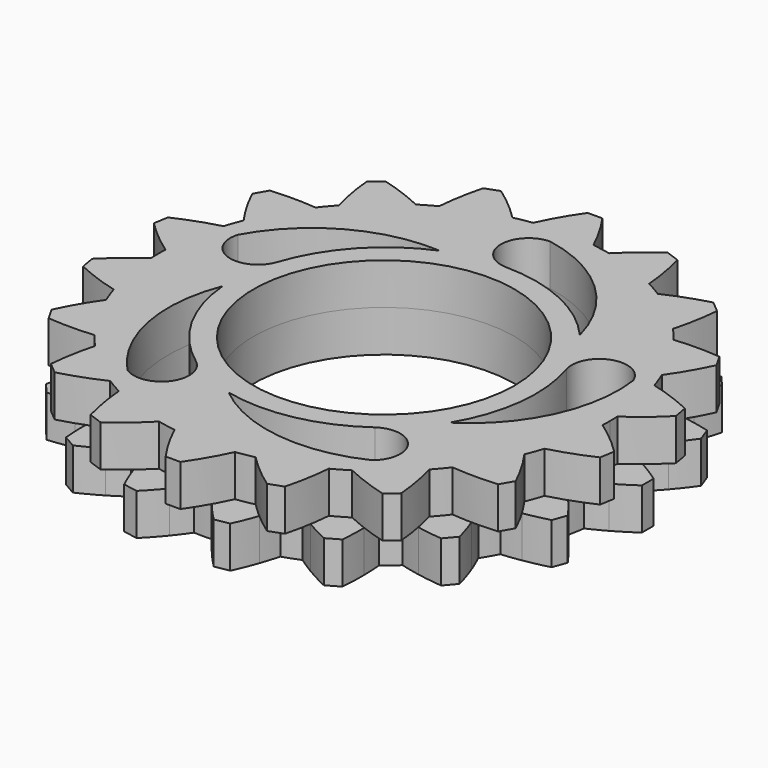
from build123d import *

# Parameters (mm, degrees)
F0_R     = 10.9982
F1_DEPTH = 3.5
F2_R     = 10.9982
F3_DEPTH = 3.5
F5_DEPTH = 25.4


with BuildPart() as f1:
    # F0 (on Top) → F1 (new body)
    with BuildSketch(Plane.XY):
        with BuildLine():
            ThreePointArc((-8.8441278606, 16.8725784154), (-6.5154837304, 17.901144426), (-4.070489347, 18.6100407435))
            ThreePointArc((-4.070489347, 18.6100407435), (-5.4892281389, 19.919494063), (-7.0197279531, 21.0963789657))
            Line((-7.0197279531, 21.0963789657), (-8.1830674177, 20.6729580282))
            ThreePointArc((-8.1830674177, 20.6729580282), (-8.5990112621, 18.7876255712), (-8.8441278606, 16.8725784154))
        make_face()
        with BuildLine():
            ThreePointArc((19.0341454654, -0.7770498061), (19.0460359539, -0.3886057666), (19.05, 0))
            ThreePointArc((19.05, 0), (19.0460359539, 0.3886057666), (19.0341454654, 0.7770498061))
            ThreePointArc((19.0341454654, 0.7770498061), (18.7605876949, 3.3079977846), (18.1520127229, 5.7798731914))
            ThreePointArc((18.1520127229, 5.7798731914), (17.901144426, 6.5154837304), (17.6204793508, 7.2402491289))
            ThreePointArc((17.6204793508, 7.2402491289), (16.4977839421, 9.525), (15.0804793508, 11.6396581802))
            ThreePointArc((15.0804793508, 11.6396581802), (14.5931466414, 12.2451039645), (14.0815233758, 12.8301675521))
            ThreePointArc((14.0815233758, 12.8301675521), (12.2451039645, 14.5931466414), (10.1900176048, 16.0955286093))
            ThreePointArc((10.1900176048, 16.0955286093), (9.525, 16.4977839421), (8.8441278606, 16.8725784154))
            ThreePointArc((8.8441278606, 16.8725784154), (6.5154837304, 17.901144426), (4.070489347, 18.6100407435))
            ThreePointArc((4.070489347, 18.6100407435), (3.3079977846, 18.7605876949), (2.54, 18.8799073091))
            ThreePointArc((2.54, 18.8799073091), (0, 19.05), (-2.54, 18.8799073091))
            ThreePointArc((-2.54, 18.8799073091), (-3.3079977846, 18.7605876949), (-4.070489347, 18.6100407435))
            ThreePointArc((-4.070489347, 18.6100407435), (-6.5154837304, 17.901144426), (-8.8441278606, 16.8725784154))
            ThreePointArc((-8.8441278606, 16.8725784154), (-9.525, 16.4977839421), (-10.1900176048, 16.0955286093))
            ThreePointArc((-10.1900176048, 16.0955286093), (-12.2451039645, 14.5931466414), (-14.0815233758, 12.8301675521))
            ThreePointArc((-14.0815233758, 12.8301675521), (-14.5931466414, 12.2451039645), (-15.0804793508, 11.6396581802))
            ThreePointArc((-15.0804793508, 11.6396581802), (-16.4977839421, 9.525), (-17.6204793508, 7.2402491289))
            ThreePointArc((-17.6204793508, 7.2402491289), (-17.901144426, 6.5154837304), (-18.1520127229, 5.7798731914))
            ThreePointArc((-18.1520127229, 5.7798731914), (-18.7605876949, 3.3079977846), (-19.0341454654, 0.7770498061))
            ThreePointArc((-19.0341454654, 0.7770498061), (-19.05, 0), (-19.0341454654, -0.7770498061))
            ThreePointArc((-19.0341454654, -0.7770498061), (-18.7605876949, -3.3079977846), (-18.1520127229, -5.7798731914))
            ThreePointArc((-18.1520127229, -5.7798731914), (-17.901144426, -6.5154837304), (-17.6204793508, -7.2402491289))
            ThreePointArc((-17.6204793508, -7.2402491289), (-16.4977839421, -9.525), (-15.0804793508, -11.6396581802))
            ThreePointArc((-15.0804793508, -11.6396581802), (-14.5931466414, -12.2451039645), (-14.0815233758, -12.8301675521))
            ThreePointArc((-14.0815233758, -12.8301675521), (-12.2451039645, -14.5931466414), (-10.1900176048, -16.0955286093))
            ThreePointArc((-10.1900176048, -16.0955286093), (-9.525, -16.4977839421), (-8.8441278606, -16.8725784154))
            ThreePointArc((-8.8441278606, -16.8725784154), (-6.5154837304, -17.901144426), (-4.070489347, -18.6100407435))
            ThreePointArc((-4.070489347, -18.6100407435), (-3.3079977846, -18.7605876949), (-2.54, -18.8799073091))
            ThreePointArc((-2.54, -18.8799073091), (0, -19.05), (2.54, -18.8799073091))
            ThreePointArc((2.54, -18.8799073091), (3.3079977846, -18.7605876949), (4.070489347, -18.6100407435))
            ThreePointArc((4.070489347, -18.6100407435), (6.5154837304, -17.901144426), (8.8441278606, -16.8725784154))
            ThreePointArc((8.8441278606, -16.8725784154), (9.525, -16.4977839421), (10.1900176048, -16.0955286093))
            ThreePointArc((10.1900176048, -16.0955286093), (12.2451039645, -14.5931466414), (14.0815233758, -12.8301675521))
            ThreePointArc((14.0815233758, -12.8301675521), (14.5931466414, -12.2451039645), (15.0804793508, -11.6396581802))
            ThreePointArc((15.0804793508, -11.6396581802), (16.4977839421, -9.525), (17.6204793508, -7.2402491289))
            ThreePointArc((17.6204793508, -7.2402491289), (17.901144426, -6.5154837304), (18.1520127229, -5.7798731914))
            ThreePointArc((18.1520127229, -5.7798731914), (18.7605876949, -3.3079977846), (19.0341454654, -0.7770498061))
        make_face()
        Circle(F0_R, mode=Mode.SUBTRACT)
        with BuildLine():
            ThreePointArc((-2.54, 18.8799073091), (0, 19.05), (2.54, 18.8799073091))
            ThreePointArc((2.54, 18.8799073091), (1.6546810385, 20.5956281756), (0.619, 22.225))
            Line((0.619, 22.225), (-0.619, 22.225))
            ThreePointArc((-0.619, 22.225), (-1.6546810385, 20.5956281756), (-2.54, 18.8799073091))
        make_face()
        with BuildLine():
            ThreePointArc((4.070489347, 18.6100407435), (6.5154837304, 17.901144426), (8.8441278606, 16.8725784154))
            ThreePointArc((8.8441278606, 16.8725784154), (8.5990112621, 18.7876255712), (8.1830674177, 20.6729580282))
            Line((8.1830674177, 20.6729580282), (7.0197279531, 21.0963789657))
            ThreePointArc((7.0197279531, 21.0963789657), (5.4892281389, 19.919494063), (4.070489347, 18.6100407435))
        make_face()
        with BuildLine():
            ThreePointArc((10.1900176048, 16.0955286093), (12.2451039645, 14.5931466414), (14.0815233758, 12.8301675521))
            ThreePointArc((14.0815233758, 12.8301675521), (14.5061738197, 14.713558047), (14.7601361356, 16.6274522179))
            Line((14.7601361356, 16.6274522179), (13.811773115, 17.4232232787))
            ThreePointArc((13.811773115, 17.4232232787), (11.9710553903, 16.840774986), (10.1900176048, 16.0955286093))
        make_face()
        with BuildLine():
            ThreePointArc((15.0804793508, 11.6396581802), (16.4977839421, 9.525), (17.6204793508, 7.2402491289))
            ThreePointArc((17.6204793508, 7.2402491289), (18.6636777262, 8.8648182733), (19.5569145991, 10.5764302751))
            Line((19.5569145991, 10.5764302751), (18.9379145991, 11.6485697249))
            ThreePointArc((18.9379145991, 11.6485697249), (17.0089966878, 11.7308099023), (15.0804793508, 11.6396581802))
        make_face()
        with BuildLine():
            ThreePointArc((18.1520127229, 5.7798731914), (18.7605876949, 3.3079977846), (19.0341454654, 0.7770498061))
            ThreePointArc((19.0341454654, 0.7770498061), (20.5700666525, 1.9468505852), (21.9948405327, 3.2497347495))
            Line((21.9948405327, 3.2497347495), (21.7798640887, 4.4689267478))
            ThreePointArc((21.7798640887, 4.4689267478), (19.9954019586, 5.2059360161), (18.1520127229, 5.7798731914))
        make_face()
        with BuildLine():
            ThreePointArc((21.9948405327, -3.2497347495), (20.5700666525, -1.9468505852), (19.0341454654, -0.7770498061))
            ThreePointArc((19.0341454654, -0.7770498061), (18.7605876949, -3.3079977846), (18.1520127229, -5.7798731914))
            ThreePointArc((18.1520127229, -5.7798731914), (19.9954019586, -5.2059360161), (21.7798640887, -4.4689267478))
            Line((21.7798640887, -4.4689267478), (21.9948405327, -3.2497347495))
        make_face()
        with BuildLine():
            ThreePointArc((19.5569145991, -10.5764302751), (18.6636777262, -8.8648182733), (17.6204793508, -7.2402491289))
            ThreePointArc((17.6204793508, -7.2402491289), (16.4977839421, -9.525), (15.0804793508, -11.6396581802))
            ThreePointArc((15.0804793508, -11.6396581802), (17.0089966878, -11.7308099023), (18.9379145991, -11.6485697249))
            Line((18.9379145991, -11.6485697249), (19.5569145991, -10.5764302751))
        make_face()
        with BuildLine():
            ThreePointArc((14.7601361356, -16.6274522179), (14.5061738197, -14.713558047), (14.0815233758, -12.8301675521))
            ThreePointArc((14.0815233758, -12.8301675521), (12.2451039645, -14.5931466414), (10.1900176048, -16.0955286093))
            ThreePointArc((10.1900176048, -16.0955286093), (11.9710553903, -16.840774986), (13.811773115, -17.4232232787))
            Line((13.811773115, -17.4232232787), (14.7601361356, -16.6274522179))
        make_face()
        with BuildLine():
            ThreePointArc((8.1830674177, -20.6729580282), (8.5990112621, -18.7876255712), (8.8441278606, -16.8725784154))
            ThreePointArc((8.8441278606, -16.8725784154), (6.5154837304, -17.901144426), (4.070489347, -18.6100407435))
            ThreePointArc((4.070489347, -18.6100407435), (5.4892281389, -19.919494063), (7.0197279531, -21.0963789657))
            Line((7.0197279531, -21.0963789657), (8.1830674177, -20.6729580282))
        make_face()
        with BuildLine():
            ThreePointArc((0.619, -22.225), (1.6546810385, -20.5956281756), (2.54, -18.8799073091))
            ThreePointArc((2.54, -18.8799073091), (0, -19.05), (-2.54, -18.8799073091))
            ThreePointArc((-2.54, -18.8799073091), (-1.6546810385, -20.5956281756), (-0.619, -22.225))
            Line((-0.619, -22.225), (0.619, -22.225))
        make_face()
        with BuildLine():
            ThreePointArc((-7.0197279531, -21.0963789657), (-5.4892281389, -19.919494063), (-4.070489347, -18.6100407435))
            ThreePointArc((-4.070489347, -18.6100407435), (-6.5154837304, -17.901144426), (-8.8441278606, -16.8725784154))
            ThreePointArc((-8.8441278606, -16.8725784154), (-8.5990112621, -18.7876255712), (-8.1830674177, -20.6729580282))
            Line((-8.1830674177, -20.6729580282), (-7.0197279531, -21.0963789657))
        make_face()
        with BuildLine():
            ThreePointArc((-13.811773115, -17.4232232787), (-11.9710553903, -16.840774986), (-10.1900176048, -16.0955286093))
            ThreePointArc((-10.1900176048, -16.0955286093), (-12.2451039645, -14.5931466414), (-14.0815233758, -12.8301675521))
            ThreePointArc((-14.0815233758, -12.8301675521), (-14.5061738197, -14.713558047), (-14.7601361356, -16.6274522179))
            Line((-14.7601361356, -16.6274522179), (-13.811773115, -17.4232232787))
        make_face()
        with BuildLine():
            ThreePointArc((-18.9379145991, -11.6485697249), (-17.0089966878, -11.7308099023), (-15.0804793508, -11.6396581802))
            ThreePointArc((-15.0804793508, -11.6396581802), (-16.4977839421, -9.525), (-17.6204793508, -7.2402491289))
            ThreePointArc((-17.6204793508, -7.2402491289), (-18.6636777262, -8.8648182733), (-19.5569145991, -10.5764302751))
            Line((-19.5569145991, -10.5764302751), (-18.9379145991, -11.6485697249))
        make_face()
        with BuildLine():
            ThreePointArc((-21.7798640887, -4.4689267478), (-19.9954019586, -5.2059360161), (-18.1520127229, -5.7798731914))
            ThreePointArc((-18.1520127229, -5.7798731914), (-18.7605876949, -3.3079977846), (-19.0341454654, -0.7770498061))
            ThreePointArc((-19.0341454654, -0.7770498061), (-20.5700666525, -1.9468505852), (-21.9948405327, -3.2497347495))
            Line((-21.9948405327, -3.2497347495), (-21.7798640887, -4.4689267478))
        make_face()
        with BuildLine():
            ThreePointArc((-19.0341454654, 0.7770498061), (-18.7605876949, 3.3079977846), (-18.1520127229, 5.7798731914))
            ThreePointArc((-18.1520127229, 5.7798731914), (-19.9954019586, 5.2059360161), (-21.7798640887, 4.4689267478))
            Line((-21.7798640887, 4.4689267478), (-21.9948405327, 3.2497347495))
            ThreePointArc((-21.9948405327, 3.2497347495), (-20.5700666525, 1.9468505852), (-19.0341454654, 0.7770498061))
        make_face()
        with BuildLine():
            ThreePointArc((-17.6204793508, 7.2402491289), (-16.4977839421, 9.525), (-15.0804793508, 11.6396581802))
            ThreePointArc((-15.0804793508, 11.6396581802), (-17.0089966878, 11.7308099023), (-18.9379145991, 11.6485697249))
            Line((-18.9379145991, 11.6485697249), (-19.5569145991, 10.5764302751))
            ThreePointArc((-19.5569145991, 10.5764302751), (-18.6636777262, 8.8648182733), (-17.6204793508, 7.2402491289))
        make_face()
        with BuildLine():
            ThreePointArc((-14.0815233758, 12.8301675521), (-12.2451039645, 14.5931466414), (-10.1900176048, 16.0955286093))
            ThreePointArc((-10.1900176048, 16.0955286093), (-11.9710553903, 16.840774986), (-13.811773115, 17.4232232787))
            Line((-13.811773115, 17.4232232787), (-14.7601361356, 16.6274522179))
            ThreePointArc((-14.7601361356, 16.6274522179), (-14.5061738197, 14.713558047), (-14.0815233758, 12.8301675521))
        make_face()
    extrude(amount=F1_DEPTH)


with BuildPart() as f3:
    # F2 (on face) → F3 (new body)
    with BuildSketch(Plane(origin=(0, 0, 0), x_dir=(1, 0, 0), z_dir=(0, 0, -1))):
        with BuildLine():
            ThreePointArc((-4.070489347, 18.6100407435), (-3.3079977846, 18.7605876949), (-2.54, 18.8799073091))
            ThreePointArc((-2.54, 18.8799073091), (-2.1755909563, 19.6325616186), (-1.7821855432, 20.3704739723))
            ThreePointArc((-1.7821855432, 20.3704739723), (-2.495270167, 21.2013498084), (-3.2497347495, 21.9948405327))
            Line((-3.2497347495, 21.9948405327), (-4.4689267478, 21.7798640887))
            ThreePointArc((-4.4689267478, 21.7798640887), (-4.9065017373, 20.7761846258), (-5.2924058238, 19.7515274286))
            ThreePointArc((-5.2924058238, 19.7515274286), (-4.6703447712, 19.1926692108), (-4.070489347, 18.6100407435))
        make_face()
        with BuildLine():
            ThreePointArc((-1.7821855432, 20.3704739723), (-2.1755909563, 19.6325616186), (-2.54, 18.8799073091))
            ThreePointArc((-2.54, 18.8799073091), (-1.6603168993, 18.9775089986), (-0.7770498061, 19.0341454654))
            ThreePointArc((-0.7770498061, 19.0341454654), (-1.2666197069, 19.7120862984), (-1.7821855432, 20.3704739723))
        make_face()
        with BuildLine():
            ThreePointArc((-0.7770498061, 19.0341454654), (-1.6603168993, 18.9775089986), (-2.54, 18.8799073091))
            ThreePointArc((-2.54, 18.8799073091), (-3.3079977846, 18.7605876949), (-4.070489347, 18.6100407435))
            ThreePointArc((-4.070489347, 18.6100407435), (-4.9305028092, 18.4008869908), (-5.7798731914, 18.1520127229))
            ThreePointArc((-5.7798731914, 18.1520127229), (-6.5154837304, 17.901144426), (-7.2402491289, 17.6204793508))
            ThreePointArc((-7.2402491289, 17.6204793508), (-8.0508778862, 17.265163343), (-8.8441278606, 16.8725784154))
            ThreePointArc((-8.8441278606, 16.8725784154), (-9.525, 16.4977839421), (-10.1900176048, 16.0955286093))
            ThreePointArc((-10.1900176048, 16.0955286093), (-10.9266311125, 15.6048464437), (-11.6396581802, 15.0804793508))
            ThreePointArc((-11.6396581802, 15.0804793508), (-12.2451039645, 14.5931466414), (-12.8301675521, 14.0815233758))
            ThreePointArc((-12.8301675521, 14.0815233758), (-13.4703841816, 13.4703841816), (-14.0815233758, 12.8301675521))
            ThreePointArc((-14.0815233758, 12.8301675521), (-14.5931466414, 12.2451039645), (-15.0804793508, 11.6396581802))
            ThreePointArc((-15.0804793508, 11.6396581802), (-15.6048464437, 10.9266311125), (-16.0955286093, 10.1900176048))
            ThreePointArc((-16.0955286093, 10.1900176048), (-16.4977839421, 9.525), (-16.8725784154, 8.8441278606))
            ThreePointArc((-16.8725784154, 8.8441278606), (-17.265163343, 8.0508778862), (-17.6204793508, 7.2402491289))
            ThreePointArc((-17.6204793508, 7.2402491289), (-17.901144426, 6.5154837304), (-18.1520127229, 5.7798731914))
            ThreePointArc((-18.1520127229, 5.7798731914), (-18.4008869908, 4.9305028092), (-18.6100407435, 4.070489347))
            ThreePointArc((-18.6100407435, 4.070489347), (-18.7605876949, 3.3079977846), (-18.8799073091, 2.54))
            ThreePointArc((-18.8799073091, 2.54), (-18.9775089986, 1.6603168993), (-19.0341454654, 0.7770498061))
            ThreePointArc((-19.0341454654, 0.7770498061), (-19.05, 0), (-19.0341454654, -0.7770498061))
            ThreePointArc((-19.0341454654, -0.7770498061), (-18.9775089986, -1.6603168993), (-18.8799073091, -2.54))
            ThreePointArc((-18.8799073091, -2.54), (-18.7605876949, -3.3079977846), (-18.6100407435, -4.070489347))
            ThreePointArc((-18.6100407435, -4.070489347), (-18.4008869908, -4.9305028092), (-18.1520127229, -5.7798731914))
            ThreePointArc((-18.1520127229, -5.7798731914), (-17.901144426, -6.5154837304), (-17.6204793508, -7.2402491289))
            ThreePointArc((-17.6204793508, -7.2402491289), (-17.265163343, -8.0508778862), (-16.8725784154, -8.8441278606))
            ThreePointArc((-16.8725784154, -8.8441278606), (-16.4977839421, -9.525), (-16.0955286093, -10.1900176048))
            ThreePointArc((-16.0955286093, -10.1900176048), (-15.6048464437, -10.9266311125), (-15.0804793508, -11.6396581802))
            ThreePointArc((-15.0804793508, -11.6396581802), (-14.5931466414, -12.2451039645), (-14.0815233758, -12.8301675521))
            ThreePointArc((-14.0815233758, -12.8301675521), (-13.4703841816, -13.4703841816), (-12.8301675521, -14.0815233758))
            ThreePointArc((-12.8301675521, -14.0815233758), (-12.2451039645, -14.5931466414), (-11.6396581802, -15.0804793508))
            ThreePointArc((-11.6396581802, -15.0804793508), (-10.9266311125, -15.6048464437), (-10.1900176048, -16.0955286093))
            ThreePointArc((-10.1900176048, -16.0955286093), (-9.525, -16.4977839421), (-8.8441278606, -16.8725784154))
            ThreePointArc((-8.8441278606, -16.8725784154), (-8.0508778862, -17.265163343), (-7.2402491289, -17.6204793508))
            ThreePointArc((-7.2402491289, -17.6204793508), (-6.5154837304, -17.901144426), (-5.7798731914, -18.1520127229))
            ThreePointArc((-5.7798731914, -18.1520127229), (-4.9305028092, -18.4008869908), (-4.070489347, -18.6100407435))
            ThreePointArc((-4.070489347, -18.6100407435), (-3.3079977846, -18.7605876949), (-2.54, -18.8799073091))
            ThreePointArc((-2.54, -18.8799073091), (-1.6603168993, -18.9775089986), (-0.7770498061, -19.0341454654))
            ThreePointArc((-0.7770498061, -19.0341454654), (0, -19.05), (0.7770498061, -19.0341454654))
            ThreePointArc((0.7770498061, -19.0341454654), (1.6603168993, -18.9775089986), (2.54, -18.8799073091))
            ThreePointArc((2.54, -18.8799073091), (3.3079977846, -18.7605876949), (4.070489347, -18.6100407435))
            ThreePointArc((4.070489347, -18.6100407435), (4.9305028092, -18.4008869908), (5.7798731914, -18.1520127229))
            ThreePointArc((5.7798731914, -18.1520127229), (6.5154837304, -17.901144426), (7.2402491289, -17.6204793508))
            ThreePointArc((7.2402491289, -17.6204793508), (8.0508778862, -17.265163343), (8.8441278606, -16.8725784154))
            ThreePointArc((8.8441278606, -16.8725784154), (9.525, -16.4977839421), (10.1900176048, -16.0955286093))
            ThreePointArc((10.1900176048, -16.0955286093), (10.9266311125, -15.6048464437), (11.6396581802, -15.0804793508))
            ThreePointArc((11.6396581802, -15.0804793508), (12.2451039645, -14.5931466414), (12.8301675521, -14.0815233758))
            ThreePointArc((12.8301675521, -14.0815233758), (13.4703841816, -13.4703841816), (14.0815233758, -12.8301675521))
            ThreePointArc((14.0815233758, -12.8301675521), (14.5931466414, -12.2451039645), (15.0804793508, -11.6396581802))
            ThreePointArc((15.0804793508, -11.6396581802), (15.6048464437, -10.9266311125), (16.0955286093, -10.1900176048))
            ThreePointArc((16.0955286093, -10.1900176048), (16.4977839421, -9.525), (16.8725784154, -8.8441278606))
            ThreePointArc((16.8725784154, -8.8441278606), (17.265163343, -8.0508778862), (17.6204793508, -7.2402491289))
            ThreePointArc((17.6204793508, -7.2402491289), (17.901144426, -6.5154837304), (18.1520127229, -5.7798731914))
            ThreePointArc((18.1520127229, -5.7798731914), (18.4008869908, -4.9305028092), (18.6100407435, -4.070489347))
            ThreePointArc((18.6100407435, -4.070489347), (18.7605876949, -3.3079977846), (18.8799073091, -2.54))
            ThreePointArc((18.8799073091, -2.54), (18.9775089986, -1.6603168993), (19.0341454654, -0.7770498061))
            ThreePointArc((19.0341454654, -0.7770498061), (19.0460359539, -0.3886057666), (19.05, 0))
            ThreePointArc((19.05, 0), (19.0460359539, 0.3886057666), (19.0341454654, 0.7770498061))
            ThreePointArc((19.0341454654, 0.7770498061), (18.9775089986, 1.6603168993), (18.8799073091, 2.54))
            ThreePointArc((18.8799073091, 2.54), (18.7605876949, 3.3079977846), (18.6100407435, 4.070489347))
            ThreePointArc((18.6100407435, 4.070489347), (18.4008869908, 4.9305028092), (18.1520127229, 5.7798731914))
            ThreePointArc((18.1520127229, 5.7798731914), (17.901144426, 6.5154837304), (17.6204793508, 7.2402491289))
            ThreePointArc((17.6204793508, 7.2402491289), (17.265163343, 8.0508778862), (16.8725784154, 8.8441278606))
            ThreePointArc((16.8725784154, 8.8441278606), (16.4977839421, 9.525), (16.0955286093, 10.1900176048))
            ThreePointArc((16.0955286093, 10.1900176048), (15.6048464437, 10.9266311125), (15.0804793508, 11.6396581802))
            ThreePointArc((15.0804793508, 11.6396581802), (14.5931466414, 12.2451039645), (14.0815233758, 12.8301675521))
            ThreePointArc((14.0815233758, 12.8301675521), (13.4703841816, 13.4703841816), (12.8301675521, 14.0815233758))
            ThreePointArc((12.8301675521, 14.0815233758), (12.2451039645, 14.5931466414), (11.6396581802, 15.0804793508))
            ThreePointArc((11.6396581802, 15.0804793508), (10.9266311125, 15.6048464437), (10.1900176048, 16.0955286093))
            ThreePointArc((10.1900176048, 16.0955286093), (9.525, 16.4977839421), (8.8441278606, 16.8725784154))
            ThreePointArc((8.8441278606, 16.8725784154), (8.0508778862, 17.265163343), (7.2402491289, 17.6204793508))
            ThreePointArc((7.2402491289, 17.6204793508), (6.5154837304, 17.901144426), (5.7798731914, 18.1520127229))
            ThreePointArc((5.7798731914, 18.1520127229), (4.9305028092, 18.4008869908), (4.070489347, 18.6100407435))
            ThreePointArc((4.070489347, 18.6100407435), (3.3079977846, 18.7605876949), (2.54, 18.8799073091))
            ThreePointArc((2.54, 18.8799073091), (1.6603168993, 18.9775089986), (0.7770498061, 19.0341454654))
            ThreePointArc((0.7770498061, 19.0341454654), (0, 19.05), (-0.7770498061, 19.0341454654))
        make_face()
        Circle(F2_R, mode=Mode.SUBTRACT)
        with BuildLine():
            ThreePointArc((-5.7798731914, 18.1520127229), (-4.9305028092, 18.4008869908), (-4.070489347, 18.6100407435))
            ThreePointArc((-4.070489347, 18.6100407435), (-4.6703447712, 19.1926692108), (-5.2924058238, 19.7515274286))
            ThreePointArc((-5.2924058238, 19.7515274286), (-5.5516973891, 18.9565114886), (-5.7798731914, 18.1520127229))
        make_face()
        with BuildLine():
            ThreePointArc((1.7821855432, 20.3704739723), (1.2666197069, 19.7120862984), (0.7770498061, 19.0341454654))
            ThreePointArc((0.7770498061, 19.0341454654), (1.6603168993, 18.9775089986), (2.54, 18.8799073091))
            ThreePointArc((2.54, 18.8799073091), (2.1755909563, 19.6325616186), (1.7821855432, 20.3704739723))
        make_face()
        with BuildLine():
            ThreePointArc((3.2497347495, 21.9948405327), (2.495270167, 21.2013498084), (1.7821855432, 20.3704739723))
            ThreePointArc((1.7821855432, 20.3704739723), (2.1755909563, 19.6325616186), (2.54, 18.8799073091))
            ThreePointArc((2.54, 18.8799073091), (3.3079977846, 18.7605876949), (4.070489347, 18.6100407435))
            ThreePointArc((4.070489347, 18.6100407435), (4.6703447712, 19.1926692108), (5.2924058238, 19.7515274286))
            ThreePointArc((5.2924058238, 19.7515274286), (4.9065017373, 20.7761846258), (4.4689267478, 21.7798640887))
            Line((4.4689267478, 21.7798640887), (3.2497347495, 21.9948405327))
        make_face()
        with BuildLine():
            ThreePointArc((-8.8441278606, 16.8725784154), (-8.0508778862, 17.265163343), (-7.2402491289, 17.6204793508))
            ThreePointArc((-7.2402491289, 17.6204793508), (-7.9321637729, 18.0900925812), (-8.6418190315, 18.5324407188))
            ThreePointArc((-8.6418190315, 18.5324407188), (-8.7591183061, 17.7044773495), (-8.8441278606, 16.8725784154))
        make_face()
        with BuildLine():
            ThreePointArc((5.2924058238, 19.7515274286), (4.6703447712, 19.1926692108), (4.070489347, 18.6100407435))
            ThreePointArc((4.070489347, 18.6100407435), (4.9305028092, 18.4008869908), (5.7798731914, 18.1520127229))
            ThreePointArc((5.7798731914, 18.1520127229), (5.5516973891, 18.9565114886), (5.2924058238, 19.7515274286))
        make_face()
        with BuildLine():
            ThreePointArc((-8.8441278606, 16.8725784154), (-8.7591183061, 17.7044773495), (-8.6418190315, 18.5324407188))
            ThreePointArc((-8.6418190315, 18.5324407188), (-9.596075663, 19.0693193055), (-10.5764302751, 19.5569145991))
            Line((-10.5764302751, 19.5569145991), (-11.6485697249, 18.9379145991))
            ThreePointArc((-11.6485697249, 18.9379145991), (-11.7164771199, 17.8451049536), (-11.7286549409, 16.7502551755))
            ThreePointArc((-11.7286549409, 16.7502551755), (-10.9529679923, 16.4378576426), (-10.1900176048, 16.0955286093))
            ThreePointArc((-10.1900176048, 16.0955286093), (-9.525, 16.4977839421), (-8.8441278606, 16.8725784154))
        make_face()
        with BuildLine():
            ThreePointArc((-11.6396581802, 15.0804793508), (-10.9266311125, 15.6048464437), (-10.1900176048, 16.0955286093))
            ThreePointArc((-10.1900176048, 16.0955286093), (-10.9529679923, 16.4378576426), (-11.7286549409, 16.7502551755))
            ThreePointArc((-11.7286549409, 16.7502551755), (-11.7003978457, 15.9145016249), (-11.6396581802, 15.0804793508))
        make_face()
        with BuildLine():
            ThreePointArc((8.6418190315, 18.5324407188), (7.9321637729, 18.0900925812), (7.2402491289, 17.6204793508))
            ThreePointArc((7.2402491289, 17.6204793508), (8.0508778862, 17.265163343), (8.8441278606, 16.8725784154))
            ThreePointArc((8.8441278606, 16.8725784154), (8.7591183061, 17.7044773495), (8.6418190315, 18.5324407188))
        make_face()
        with BuildLine():
            ThreePointArc((10.5764302751, 19.5569145991), (9.596075663, 19.0693193055), (8.6418190315, 18.5324407188))
            ThreePointArc((8.6418190315, 18.5324407188), (8.7591183061, 17.7044773495), (8.8441278606, 16.8725784154))
            ThreePointArc((8.8441278606, 16.8725784154), (9.525, 16.4977839421), (10.1900176048, 16.0955286093))
            ThreePointArc((10.1900176048, 16.0955286093), (10.9529679923, 16.4378576426), (11.7286549409, 16.7502551755))
            ThreePointArc((11.7286549409, 16.7502551755), (11.7164771199, 17.8451049536), (11.6485697249, 18.9379145991))
            Line((11.6485697249, 18.9379145991), (10.5764302751, 19.5569145991))
        make_face()
        with BuildLine():
            ThreePointArc((-14.0815233758, 12.8301675521), (-13.4703841816, 13.4703841816), (-12.8301675521, 14.0815233758))
            ThreePointArc((-12.8301675521, 14.0815233758), (-13.6409718217, 14.2861667174), (-14.4591216048, 14.4591216048))
            ThreePointArc((-14.4591216048, 14.4591216048), (-14.2861667174, 13.6409718217), (-14.0815233758, 12.8301675521))
        make_face()
        with BuildLine():
            ThreePointArc((11.7286549409, 16.7502551755), (10.9529679923, 16.4378576426), (10.1900176048, 16.0955286093))
            ThreePointArc((10.1900176048, 16.0955286093), (10.9266311125, 15.6048464437), (11.6396581802, 15.0804793508))
            ThreePointArc((11.6396581802, 15.0804793508), (11.7003978457, 15.9145016249), (11.7286549409, 16.7502551755))
        make_face()
        with BuildLine():
            ThreePointArc((-14.0815233758, 12.8301675521), (-14.2861667174, 13.6409718217), (-14.4591216048, 14.4591216048))
            ThreePointArc((-14.4591216048, 14.4591216048), (-15.539452811, 14.6372474612), (-16.6274522179, 14.7601361356))
            Line((-16.6274522179, 14.7601361356), (-17.4232232787, 13.811773115))
            ThreePointArc((-17.4232232787, 13.811773115), (-17.1132724451, 12.7616422582), (-16.7502551755, 11.7286549409))
            ThreePointArc((-16.7502551755, 11.7286549409), (-15.9145016249, 11.7003978457), (-15.0804793508, 11.6396581802))
            ThreePointArc((-15.0804793508, 11.6396581802), (-14.5931466414, 12.2451039645), (-14.0815233758, 12.8301675521))
        make_face()
        with BuildLine():
            ThreePointArc((-16.0955286093, 10.1900176048), (-15.6048464437, 10.9266311125), (-15.0804793508, 11.6396581802))
            ThreePointArc((-15.0804793508, 11.6396581802), (-15.9145016249, 11.7003978457), (-16.7502551755, 11.7286549409))
            ThreePointArc((-16.7502551755, 11.7286549409), (-16.4378576426, 10.9529679923), (-16.0955286093, 10.1900176048))
        make_face()
        with BuildLine():
            ThreePointArc((14.4591216048, 14.4591216048), (13.6409718217, 14.2861667174), (12.8301675521, 14.0815233758))
            ThreePointArc((12.8301675521, 14.0815233758), (13.4703841816, 13.4703841816), (14.0815233758, 12.8301675521))
            ThreePointArc((14.0815233758, 12.8301675521), (14.2861667174, 13.6409718217), (14.4591216048, 14.4591216048))
        make_face()
        with BuildLine():
            ThreePointArc((16.6274522179, 14.7601361356), (15.539452811, 14.6372474612), (14.4591216048, 14.4591216048))
            ThreePointArc((14.4591216048, 14.4591216048), (14.2861667174, 13.6409718217), (14.0815233758, 12.8301675521))
            ThreePointArc((14.0815233758, 12.8301675521), (14.5931466414, 12.2451039645), (15.0804793508, 11.6396581802))
            ThreePointArc((15.0804793508, 11.6396581802), (15.9145016249, 11.7003978457), (16.7502551755, 11.7286549409))
            ThreePointArc((16.7502551755, 11.7286549409), (17.1132724451, 12.7616422582), (17.4232232787, 13.811773115))
            Line((17.4232232787, 13.811773115), (16.6274522179, 14.7601361356))
        make_face()
        with BuildLine():
            ThreePointArc((-17.6204793508, 7.2402491289), (-17.265163343, 8.0508778862), (-16.8725784154, 8.8441278606))
            ThreePointArc((-16.8725784154, 8.8441278606), (-17.7044773495, 8.7591183061), (-18.5324407188, 8.6418190315))
            ThreePointArc((-18.5324407188, 8.6418190315), (-18.0900925812, 7.9321637729), (-17.6204793508, 7.2402491289))
        make_face()
        with BuildLine():
            ThreePointArc((16.7502551755, 11.7286549409), (15.9145016249, 11.7003978457), (15.0804793508, 11.6396581802))
            ThreePointArc((15.0804793508, 11.6396581802), (15.6048464437, 10.9266311125), (16.0955286093, 10.1900176048))
            ThreePointArc((16.0955286093, 10.1900176048), (16.4378576426, 10.9529679923), (16.7502551755, 11.7286549409))
        make_face()
        with BuildLine():
            ThreePointArc((-17.6204793508, 7.2402491289), (-18.0900925812, 7.9321637729), (-18.5324407188, 8.6418190315))
            ThreePointArc((-18.5324407188, 8.6418190315), (-19.6085426121, 8.4397075502), (-20.6729580282, 8.1830674177))
            Line((-20.6729580282, 8.1830674177), (-21.0963789657, 7.0197279531))
            ThreePointArc((-21.0963789657, 7.0197279531), (-20.4459545484, 6.1389371647), (-19.7515274286, 5.2924058238))
            ThreePointArc((-19.7515274286, 5.2924058238), (-18.9565114886, 5.5516973891), (-18.1520127229, 5.7798731914))
            ThreePointArc((-18.1520127229, 5.7798731914), (-17.901144426, 6.5154837304), (-17.6204793508, 7.2402491289))
        make_face()
        with BuildLine():
            ThreePointArc((-18.6100407435, 4.070489347), (-18.4008869908, 4.9305028092), (-18.1520127229, 5.7798731914))
            ThreePointArc((-18.1520127229, 5.7798731914), (-18.9565114886, 5.5516973891), (-19.7515274286, 5.2924058238))
            ThreePointArc((-19.7515274286, 5.2924058238), (-19.1926692108, 4.6703447712), (-18.6100407435, 4.070489347))
        make_face()
        with BuildLine():
            ThreePointArc((18.5324407188, 8.6418190315), (17.7044773495, 8.7591183061), (16.8725784154, 8.8441278606))
            ThreePointArc((16.8725784154, 8.8441278606), (17.265163343, 8.0508778862), (17.6204793508, 7.2402491289))
            ThreePointArc((17.6204793508, 7.2402491289), (18.0900925812, 7.9321637729), (18.5324407188, 8.6418190315))
        make_face()
        with BuildLine():
            ThreePointArc((20.6729580282, 8.1830674177), (19.6085426121, 8.4397075502), (18.5324407188, 8.6418190315))
            ThreePointArc((18.5324407188, 8.6418190315), (18.0900925812, 7.9321637729), (17.6204793508, 7.2402491289))
            ThreePointArc((17.6204793508, 7.2402491289), (17.901144426, 6.5154837304), (18.1520127229, 5.7798731914))
            ThreePointArc((18.1520127229, 5.7798731914), (18.9565114886, 5.5516973891), (19.7515274286, 5.2924058238))
            ThreePointArc((19.7515274286, 5.2924058238), (20.4459545484, 6.1389371647), (21.0963789657, 7.0197279531))
            Line((21.0963789657, 7.0197279531), (20.6729580282, 8.1830674177))
        make_face()
        with BuildLine():
            ThreePointArc((-19.0341454654, 0.7770498061), (-18.9775089986, 1.6603168993), (-18.8799073091, 2.54))
            ThreePointArc((-18.8799073091, 2.54), (-19.6325616186, 2.1755909563), (-20.3704739723, 1.7821855432))
            ThreePointArc((-20.3704739723, 1.7821855432), (-19.7120862984, 1.2666197069), (-19.0341454654, 0.7770498061))
        make_face()
        with BuildLine():
            ThreePointArc((19.7515274286, 5.2924058238), (18.9565114886, 5.5516973891), (18.1520127229, 5.7798731914))
            ThreePointArc((18.1520127229, 5.7798731914), (18.4008869908, 4.9305028092), (18.6100407435, 4.070489347))
            ThreePointArc((18.6100407435, 4.070489347), (19.1926692108, 4.6703447712), (19.7515274286, 5.2924058238))
        make_face()
        with BuildLine():
            ThreePointArc((-19.0341454654, 0.7770498061), (-19.7120862984, 1.2666197069), (-20.3704739723, 1.7821855432))
            ThreePointArc((-20.3704739723, 1.7821855432), (-21.3125527829, 1.2242143519), (-22.225, 0.619))
            Line((-22.225, 0.619), (-22.225, -0.619))
            ThreePointArc((-22.225, -0.619), (-21.3125527829, -1.2242143519), (-20.3704739723, -1.7821855432))
            ThreePointArc((-20.3704739723, -1.7821855432), (-19.7120862984, -1.2666197069), (-19.0341454654, -0.7770498061))
            ThreePointArc((-19.0341454654, -0.7770498061), (-19.05, 0), (-19.0341454654, 0.7770498061))
        make_face()
        with BuildLine():
            ThreePointArc((-18.8799073091, -2.54), (-18.9775089986, -1.6603168993), (-19.0341454654, -0.7770498061))
            ThreePointArc((-19.0341454654, -0.7770498061), (-19.7120862984, -1.2666197069), (-20.3704739723, -1.7821855432))
            ThreePointArc((-20.3704739723, -1.7821855432), (-19.6325616186, -2.1755909563), (-18.8799073091, -2.54))
        make_face()
        with BuildLine():
            ThreePointArc((20.3704739723, 1.7821855432), (19.6325616186, 2.1755909563), (18.8799073091, 2.54))
            ThreePointArc((18.8799073091, 2.54), (18.9775089986, 1.6603168993), (19.0341454654, 0.7770498061))
            ThreePointArc((19.0341454654, 0.7770498061), (19.7120862984, 1.2666197069), (20.3704739723, 1.7821855432))
        make_face()
        with BuildLine():
            ThreePointArc((22.225, 0.619), (21.3125527829, 1.2242143519), (20.3704739723, 1.7821855432))
            ThreePointArc((20.3704739723, 1.7821855432), (19.7120862984, 1.2666197069), (19.0341454654, 0.7770498061))
            ThreePointArc((19.0341454654, 0.7770498061), (19.0460359539, 0.3886057666), (19.05, 0))
            ThreePointArc((19.05, 0), (19.0460359539, -0.3886057666), (19.0341454654, -0.7770498061))
            ThreePointArc((19.0341454654, -0.7770498061), (19.7120862984, -1.2666197069), (20.3704739723, -1.7821855432))
            ThreePointArc((20.3704739723, -1.7821855432), (21.3125527829, -1.2242143519), (22.225, -0.619))
            Line((22.225, -0.619), (22.225, 0.619))
        make_face()
        with BuildLine():
            ThreePointArc((-18.1520127229, -5.7798731914), (-18.4008869908, -4.9305028092), (-18.6100407435, -4.070489347))
            ThreePointArc((-18.6100407435, -4.070489347), (-19.1926692108, -4.6703447712), (-19.7515274286, -5.2924058238))
            ThreePointArc((-19.7515274286, -5.2924058238), (-18.9565114886, -5.5516973891), (-18.1520127229, -5.7798731914))
        make_face()
        with BuildLine():
            ThreePointArc((-18.1520127229, -5.7798731914), (-18.9565114886, -5.5516973891), (-19.7515274286, -5.2924058238))
            ThreePointArc((-19.7515274286, -5.2924058238), (-20.4459545484, -6.1389371647), (-21.0963789657, -7.0197279531))
            Line((-21.0963789657, -7.0197279531), (-20.6729580282, -8.1830674177))
            ThreePointArc((-20.6729580282, -8.1830674177), (-19.6085426121, -8.4397075502), (-18.5324407188, -8.6418190315))
            ThreePointArc((-18.5324407188, -8.6418190315), (-18.0900925812, -7.9321637729), (-17.6204793508, -7.2402491289))
            ThreePointArc((-17.6204793508, -7.2402491289), (-17.901144426, -6.5154837304), (-18.1520127229, -5.7798731914))
        make_face()
        with BuildLine():
            ThreePointArc((20.3704739723, -1.7821855432), (19.7120862984, -1.2666197069), (19.0341454654, -0.7770498061))
            ThreePointArc((19.0341454654, -0.7770498061), (18.9775089986, -1.6603168993), (18.8799073091, -2.54))
            ThreePointArc((18.8799073091, -2.54), (19.6325616186, -2.1755909563), (20.3704739723, -1.7821855432))
        make_face()
        with BuildLine():
            ThreePointArc((-16.8725784154, -8.8441278606), (-17.265163343, -8.0508778862), (-17.6204793508, -7.2402491289))
            ThreePointArc((-17.6204793508, -7.2402491289), (-18.0900925812, -7.9321637729), (-18.5324407188, -8.6418190315))
            ThreePointArc((-18.5324407188, -8.6418190315), (-17.7044773495, -8.7591183061), (-16.8725784154, -8.8441278606))
        make_face()
        with BuildLine():
            ThreePointArc((19.7515274286, -5.2924058238), (19.1926692108, -4.6703447712), (18.6100407435, -4.070489347))
            ThreePointArc((18.6100407435, -4.070489347), (18.4008869908, -4.9305028092), (18.1520127229, -5.7798731914))
            ThreePointArc((18.1520127229, -5.7798731914), (18.9565114886, -5.5516973891), (19.7515274286, -5.2924058238))
        make_face()
        with BuildLine():
            ThreePointArc((-15.0804793508, -11.6396581802), (-15.6048464437, -10.9266311125), (-16.0955286093, -10.1900176048))
            ThreePointArc((-16.0955286093, -10.1900176048), (-16.4378576426, -10.9529679923), (-16.7502551755, -11.7286549409))
            ThreePointArc((-16.7502551755, -11.7286549409), (-15.9145016249, -11.7003978457), (-15.0804793508, -11.6396581802))
        make_face()
        with BuildLine():
            ThreePointArc((21.0963789657, -7.0197279531), (20.4459545484, -6.1389371647), (19.7515274286, -5.2924058238))
            ThreePointArc((19.7515274286, -5.2924058238), (18.9565114886, -5.5516973891), (18.1520127229, -5.7798731914))
            ThreePointArc((18.1520127229, -5.7798731914), (17.901144426, -6.5154837304), (17.6204793508, -7.2402491289))
            ThreePointArc((17.6204793508, -7.2402491289), (18.0900925812, -7.9321637729), (18.5324407188, -8.6418190315))
            ThreePointArc((18.5324407188, -8.6418190315), (19.6085426121, -8.4397075502), (20.6729580282, -8.1830674177))
            Line((20.6729580282, -8.1830674177), (21.0963789657, -7.0197279531))
        make_face()
        with BuildLine():
            ThreePointArc((-15.0804793508, -11.6396581802), (-15.9145016249, -11.7003978457), (-16.7502551755, -11.7286549409))
            ThreePointArc((-16.7502551755, -11.7286549409), (-17.1132724451, -12.7616422582), (-17.4232232787, -13.811773115))
            Line((-17.4232232787, -13.811773115), (-16.6274522179, -14.7601361356))
            ThreePointArc((-16.6274522179, -14.7601361356), (-15.539452811, -14.6372474612), (-14.4591216048, -14.4591216048))
            ThreePointArc((-14.4591216048, -14.4591216048), (-14.2861667174, -13.6409718217), (-14.0815233758, -12.8301675521))
            ThreePointArc((-14.0815233758, -12.8301675521), (-14.5931466414, -12.2451039645), (-15.0804793508, -11.6396581802))
        make_face()
        with BuildLine():
            ThreePointArc((18.5324407188, -8.6418190315), (18.0900925812, -7.9321637729), (17.6204793508, -7.2402491289))
            ThreePointArc((17.6204793508, -7.2402491289), (17.265163343, -8.0508778862), (16.8725784154, -8.8441278606))
            ThreePointArc((16.8725784154, -8.8441278606), (17.7044773495, -8.7591183061), (18.5324407188, -8.6418190315))
        make_face()
        with BuildLine():
            ThreePointArc((-12.8301675521, -14.0815233758), (-13.4703841816, -13.4703841816), (-14.0815233758, -12.8301675521))
            ThreePointArc((-14.0815233758, -12.8301675521), (-14.2861667174, -13.6409718217), (-14.4591216048, -14.4591216048))
            ThreePointArc((-14.4591216048, -14.4591216048), (-13.6409718217, -14.2861667174), (-12.8301675521, -14.0815233758))
        make_face()
        with BuildLine():
            ThreePointArc((16.7502551755, -11.7286549409), (16.4378576426, -10.9529679923), (16.0955286093, -10.1900176048))
            ThreePointArc((16.0955286093, -10.1900176048), (15.6048464437, -10.9266311125), (15.0804793508, -11.6396581802))
            ThreePointArc((15.0804793508, -11.6396581802), (15.9145016249, -11.7003978457), (16.7502551755, -11.7286549409))
        make_face()
        with BuildLine():
            ThreePointArc((-10.1900176048, -16.0955286093), (-10.9266311125, -15.6048464437), (-11.6396581802, -15.0804793508))
            ThreePointArc((-11.6396581802, -15.0804793508), (-11.7003978457, -15.9145016249), (-11.7286549409, -16.7502551755))
            ThreePointArc((-11.7286549409, -16.7502551755), (-10.9529679923, -16.4378576426), (-10.1900176048, -16.0955286093))
        make_face()
        with BuildLine():
            ThreePointArc((17.4232232787, -13.811773115), (17.1132724451, -12.7616422582), (16.7502551755, -11.7286549409))
            ThreePointArc((16.7502551755, -11.7286549409), (15.9145016249, -11.7003978457), (15.0804793508, -11.6396581802))
            ThreePointArc((15.0804793508, -11.6396581802), (14.5931466414, -12.2451039645), (14.0815233758, -12.8301675521))
            ThreePointArc((14.0815233758, -12.8301675521), (14.2861667174, -13.6409718217), (14.4591216048, -14.4591216048))
            ThreePointArc((14.4591216048, -14.4591216048), (15.539452811, -14.6372474612), (16.6274522179, -14.7601361356))
            Line((16.6274522179, -14.7601361356), (17.4232232787, -13.811773115))
        make_face()
        with BuildLine():
            ThreePointArc((-10.1900176048, -16.0955286093), (-10.9529679923, -16.4378576426), (-11.7286549409, -16.7502551755))
            ThreePointArc((-11.7286549409, -16.7502551755), (-11.7164771199, -17.8451049536), (-11.6485697249, -18.9379145991))
            Line((-11.6485697249, -18.9379145991), (-10.5764302751, -19.5569145991))
            ThreePointArc((-10.5764302751, -19.5569145991), (-9.596075663, -19.0693193055), (-8.6418190315, -18.5324407188))
            ThreePointArc((-8.6418190315, -18.5324407188), (-8.7591183061, -17.7044773495), (-8.8441278606, -16.8725784154))
            ThreePointArc((-8.8441278606, -16.8725784154), (-9.525, -16.4977839421), (-10.1900176048, -16.0955286093))
        make_face()
        with BuildLine():
            ThreePointArc((14.4591216048, -14.4591216048), (14.2861667174, -13.6409718217), (14.0815233758, -12.8301675521))
            ThreePointArc((14.0815233758, -12.8301675521), (13.4703841816, -13.4703841816), (12.8301675521, -14.0815233758))
            ThreePointArc((12.8301675521, -14.0815233758), (13.6409718217, -14.2861667174), (14.4591216048, -14.4591216048))
        make_face()
        with BuildLine():
            ThreePointArc((-7.2402491289, -17.6204793508), (-8.0508778862, -17.265163343), (-8.8441278606, -16.8725784154))
            ThreePointArc((-8.8441278606, -16.8725784154), (-8.7591183061, -17.7044773495), (-8.6418190315, -18.5324407188))
            ThreePointArc((-8.6418190315, -18.5324407188), (-7.9321637729, -18.0900925812), (-7.2402491289, -17.6204793508))
        make_face()
        with BuildLine():
            ThreePointArc((11.7286549409, -16.7502551755), (11.7003978457, -15.9145016249), (11.6396581802, -15.0804793508))
            ThreePointArc((11.6396581802, -15.0804793508), (10.9266311125, -15.6048464437), (10.1900176048, -16.0955286093))
            ThreePointArc((10.1900176048, -16.0955286093), (10.9529679923, -16.4378576426), (11.7286549409, -16.7502551755))
        make_face()
        with BuildLine():
            ThreePointArc((-4.070489347, -18.6100407435), (-4.9305028092, -18.4008869908), (-5.7798731914, -18.1520127229))
            ThreePointArc((-5.7798731914, -18.1520127229), (-5.5516973891, -18.9565114886), (-5.2924058238, -19.7515274286))
            ThreePointArc((-5.2924058238, -19.7515274286), (-4.6703447712, -19.1926692108), (-4.070489347, -18.6100407435))
        make_face()
        with BuildLine():
            ThreePointArc((11.6485697249, -18.9379145991), (11.7164771199, -17.8451049536), (11.7286549409, -16.7502551755))
            ThreePointArc((11.7286549409, -16.7502551755), (10.9529679923, -16.4378576426), (10.1900176048, -16.0955286093))
            ThreePointArc((10.1900176048, -16.0955286093), (9.525, -16.4977839421), (8.8441278606, -16.8725784154))
            ThreePointArc((8.8441278606, -16.8725784154), (8.7591183061, -17.7044773495), (8.6418190315, -18.5324407188))
            ThreePointArc((8.6418190315, -18.5324407188), (9.596075663, -19.0693193055), (10.5764302751, -19.5569145991))
            Line((10.5764302751, -19.5569145991), (11.6485697249, -18.9379145991))
        make_face()
        with BuildLine():
            ThreePointArc((-4.070489347, -18.6100407435), (-4.6703447712, -19.1926692108), (-5.2924058238, -19.7515274286))
            ThreePointArc((-5.2924058238, -19.7515274286), (-4.9065017373, -20.7761846258), (-4.4689267478, -21.7798640887))
            Line((-4.4689267478, -21.7798640887), (-3.2497347495, -21.9948405327))
            ThreePointArc((-3.2497347495, -21.9948405327), (-2.495270167, -21.2013498084), (-1.7821855432, -20.3704739723))
            ThreePointArc((-1.7821855432, -20.3704739723), (-2.1755909563, -19.6325616186), (-2.54, -18.8799073091))
            ThreePointArc((-2.54, -18.8799073091), (-3.3079977846, -18.7605876949), (-4.070489347, -18.6100407435))
        make_face()
        with BuildLine():
            ThreePointArc((8.6418190315, -18.5324407188), (8.7591183061, -17.7044773495), (8.8441278606, -16.8725784154))
            ThreePointArc((8.8441278606, -16.8725784154), (8.0508778862, -17.265163343), (7.2402491289, -17.6204793508))
            ThreePointArc((7.2402491289, -17.6204793508), (7.9321637729, -18.0900925812), (8.6418190315, -18.5324407188))
        make_face()
        with BuildLine():
            ThreePointArc((-0.7770498061, -19.0341454654), (-1.6603168993, -18.9775089986), (-2.54, -18.8799073091))
            ThreePointArc((-2.54, -18.8799073091), (-2.1755909563, -19.6325616186), (-1.7821855432, -20.3704739723))
            ThreePointArc((-1.7821855432, -20.3704739723), (-1.2666197069, -19.7120862984), (-0.7770498061, -19.0341454654))
        make_face()
        with BuildLine():
            ThreePointArc((2.54, -18.8799073091), (1.6603168993, -18.9775089986), (0.7770498061, -19.0341454654))
            ThreePointArc((0.7770498061, -19.0341454654), (1.2666197069, -19.7120862984), (1.7821855432, -20.3704739723))
            ThreePointArc((1.7821855432, -20.3704739723), (2.1755909563, -19.6325616186), (2.54, -18.8799073091))
        make_face()
        with BuildLine():
            ThreePointArc((4.4689267478, -21.7798640887), (4.9065017373, -20.7761846258), (5.2924058238, -19.7515274286))
            ThreePointArc((5.2924058238, -19.7515274286), (4.6703447712, -19.1926692108), (4.070489347, -18.6100407435))
            ThreePointArc((4.070489347, -18.6100407435), (3.3079977846, -18.7605876949), (2.54, -18.8799073091))
            ThreePointArc((2.54, -18.8799073091), (2.1755909563, -19.6325616186), (1.7821855432, -20.3704739723))
            ThreePointArc((1.7821855432, -20.3704739723), (2.495270167, -21.2013498084), (3.2497347495, -21.9948405327))
            Line((3.2497347495, -21.9948405327), (4.4689267478, -21.7798640887))
        make_face()
    extrude(amount=F3_DEPTH)


with BuildPart() as f5_tool:
    # F4 (on face) → F5 (new body)
    with BuildSketch(Plane.XY.offset(3.5)):
        with BuildLine():
            ThreePointArc((-4.8632466447, 11.9354155686), (-11.7061563249, 10.3882690214), (-16.6490161261, 5.4095932623))
            ThreePointArc((-16.6490161261, 5.4095932623), (-15.1317445211, 2.5139242312), (-12.2022144556, 3.9647398143))
            ThreePointArc((-12.2022144556, 3.9647398143), (-9.394216897, 8.7432877986), (-4.8632466447, 11.9354155686))
        make_face()
        with BuildLine():
            ThreePointArc((0, 12.8301675521), (5.4123881646, 11.6362557119), (9.8484288901, 8.3134686574))
            ThreePointArc((9.8484288901, 8.3134686574), (6.2624297026, 14.3433679233), (0, 17.5058115274))
            ThreePointArc((0, 17.5058115274), (-2.28508219, 15.1679895398), (0, 12.8301675521))
        make_face()
        with BuildLine():
            ThreePointArc((10.9499104346, -6.7974093739), (15.5765507333, -1.5235801317), (16.6490161261, 5.4095932623))
            ThreePointArc((16.6490161261, 5.4095932623), (13.7194860606, 6.8604088453), (12.2022144556, 3.9647398143))
            ThreePointArc((12.2022144556, 3.9647398143), (12.7392567431, -1.5516862668), (10.9499104346, -6.7974093739))
        make_face()
        with BuildLine():
            ThreePointArc((-3.0810120678, -12.5144986859), (3.364408078, -15.2849922293), (10.2896578452, -14.162499026))
            ThreePointArc((10.2896578452, -14.162499026), (10.7641908836, -10.9280236966), (7.5413832716, -10.3798235904))
            ThreePointArc((7.5413832716, -10.3798235904), (2.460905494, -12.5952505647), (-3.0810120678, -12.5144986859))
        make_face()
        with BuildLine():
            ThreePointArc((-12.8540806122, -0.9369761662), (-13.497232189, -7.9230645838), (-10.2896578452, -14.162499026))
            ThreePointArc((-10.2896578452, -14.162499026), (-7.0668502332, -13.6142989197), (-7.5413832716, -10.3798235904))
            ThreePointArc((-7.5413832716, -10.3798235904), (-11.2183335047, -6.2326066789), (-12.8540806122, -0.9369761662))
        make_face()
    extrude(amount=-F5_DEPTH)


with BuildPart() as f1_1:
    add(f1.part)

    # F5: cut by f5_tool
    add(f5_tool.part, mode=Mode.SUBTRACT)


with BuildPart() as f3_1:
    add(f3.part)

    # F5: cut by f5_tool
    add(f5_tool.part, mode=Mode.SUBTRACT)


solid = Compound([f1_1.part, f3_1.part])
